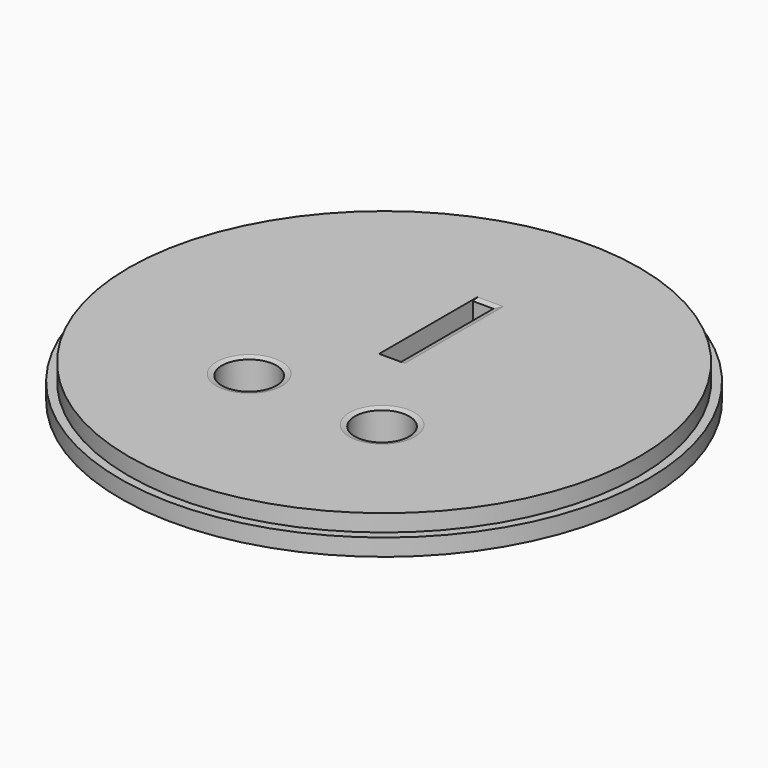
from build123d import *

# Parameters (mm, degrees)
F0_R         = 24.60625
F1_DEPTH     = 1.5875
F2_R         = 23.8125
F3_DEPTH     = 3.175
F6_W         = 1.888648374
F6_H         = 10.8168021543
F7_DEPTH     = 3.176
F5_R         = 2.54
F8_DEPTH     = 3.176
F4_R         = 2.54
F9_DEPTH     = 3.176
F10_C1_SIZE2 = 0.508
F10_C1_SIZE  = 0.1361181898
F10_C2_SIZE2 = 0.1361181898
F10_C2_SIZE  = 0.508
F10_C3_SIZE2 = 0.508
F10_C3_SIZE  = 0.1361181898
F10_C4_SIZE2 = 0.508
F10_C4_SIZE  = 0.1361181898
F11_SIZE2    = 0.1361181898
F11_SIZE     = 0.508
F12_SIZE2    = 0.1361181898
F12_SIZE     = 0.508


# Not quite as in the source:
# - a length typed as a fraction of an inch, garbled in the dataset ("3 / 203.2 mm" for 3/8 in), is restored


with BuildPart() as f1:
    # F0 (on Top) → F1 (new body)
    with BuildSketch(Plane.XY):
        Circle(F0_R)
    extrude(amount=F1_DEPTH)

    # F2 (on Top) → F3 (join)
    with BuildSketch(Plane.XY):
        Circle(F2_R)
    extrude(amount=F3_DEPTH)

    # F6 (on Top) → F7 (cut, through all)
    with BuildSketch(Plane.XY):
        with Locations((-0.156514463, 6.341986882)):
            Rectangle(F6_W, F6_H)
    extrude(amount=F7_DEPTH, mode=Mode.SUBTRACT)

    # F5 (on Top) → F8 (cut, through all)
    with BuildSketch(Plane.XY):
        with Locations((6.0491965251, -7.797766786)):
            Circle(F5_R)
    extrude(amount=F8_DEPTH, mode=Mode.SUBTRACT)

    # F4 (on Top) → F9 (cut, through all)
    with BuildSketch(Plane.XY):
        with Locations((-6.5096618418, -7.5848015673)):
            Circle(F4_R)
    extrude(amount=F9_DEPTH, mode=Mode.SUBTRACT)

    # F10: chamfer of 0.508 x 0.1361181898 on 4 edges, made by hand

    # F10_c1
    f10_c1_edges = [f1.edges().sort_by_distance(p)[0] for p in [
        (-1.10083865, 6.341986882, 0),
    ]]
    f10_c1_side = f1.faces().sort_by_distance((-1.1035610138, 6.341986882, 0))[0]
    chamfer(f10_c1_edges, length=F10_C1_SIZE, length2=F10_C1_SIZE2, reference=f10_c1_side)

    # F10_c2
    f10_c2_edges = [f1.edges().sort_by_distance(p)[0] for p in [
        (-0.156514463, 0.9335858049, 3.175),
    ]]
    f10_c2_side = f1.faces().sort_by_distance((-0.156514463, 0.9335858049, 3.1722776362))[0]
    chamfer(f10_c2_edges, length=F10_C2_SIZE, length2=F10_C2_SIZE2, reference=f10_c2_side)

    # F10_c3
    f10_c3_edges = [f1.edges().sort_by_distance(p)[0] for p in [
        (0.787809724, 6.341986882, 3.175),
    ]]
    f10_c3_side = f1.faces().sort_by_distance((0.787809724, 6.341986882, 3.1722776362))[0]
    chamfer(f10_c3_edges, length=F10_C3_SIZE, length2=F10_C3_SIZE2, reference=f10_c3_side)

    # F10_c4
    f10_c4_edges = [f1.edges().sort_by_distance(p)[0] for p in [
        (-0.156514463, 11.7503879592, 3.175),
    ]]
    f10_c4_side = f1.faces().sort_by_distance((-0.156514463, 11.7503879592, 3.1722776362))[0]
    chamfer(f10_c4_edges, length=F10_C4_SIZE, length2=F10_C4_SIZE2, reference=f10_c4_side)

    # F11
    f11_edges = [f1.edges().sort_by_distance(p)[0] for p in [
        (-9.049662, -7.584802, 3.175),
    ]]
    chamfer(f11_edges, length=F11_SIZE, length2=F11_SIZE2)

    # F12
    f12_edges = [f1.edges().sort_by_distance(p)[0] for p in [
        (3.509197, -7.797767, 3.175),
    ]]
    chamfer(f12_edges, length=F12_SIZE, length2=F12_SIZE2)


solid = f1.part
